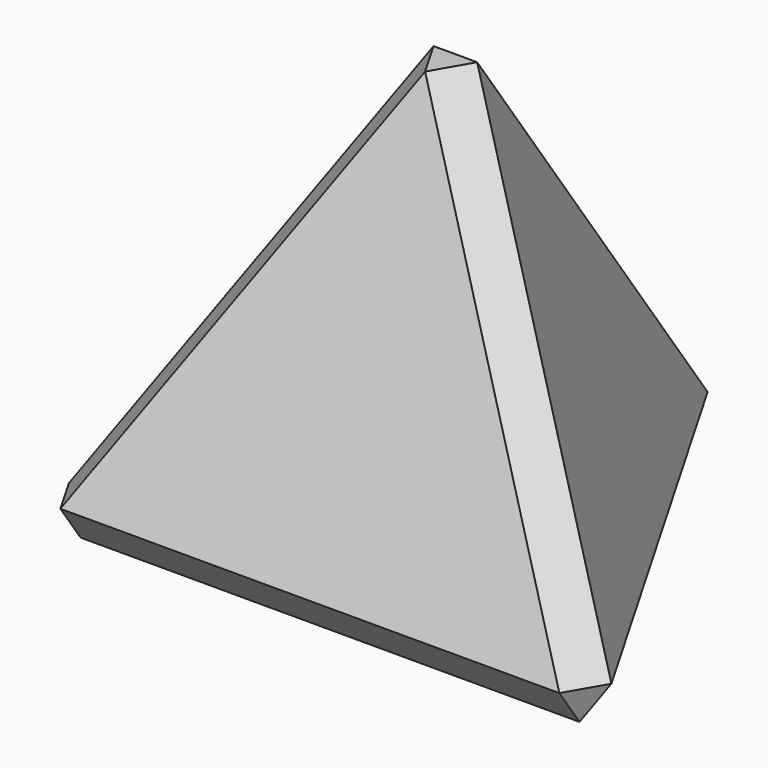
from build123d import *

# Parameters (mm, degrees)
F4_SIZE = 2.4


with BuildPart() as f3:
    # F0 (on Top) → F3 section 0
    with BuildSketch(Plane.XY, mode=Mode.PRIVATE) as f3_s0:
        Polygon((20, -11.5470053838), (0, 23.0940107676), (-20, -11.5470053838), align=None)
    loft([f3_s0.sketch, Vertex(0, 0, 32.66)])

    # F4
    f4_edges = [f3.edges().sort_by_distance(p)[0] for p in [
        (0, -11.547005, 0),
        (-10, 5.773503, 0),
        (10, 5.773503, 0),
        (10, -5.773503, 16.33),
        (-10, -5.773503, 16.33),
        (0, 11.547005, 16.33),
    ]]
    chamfer(f4_edges, length=F4_SIZE)


solid = f3.part
